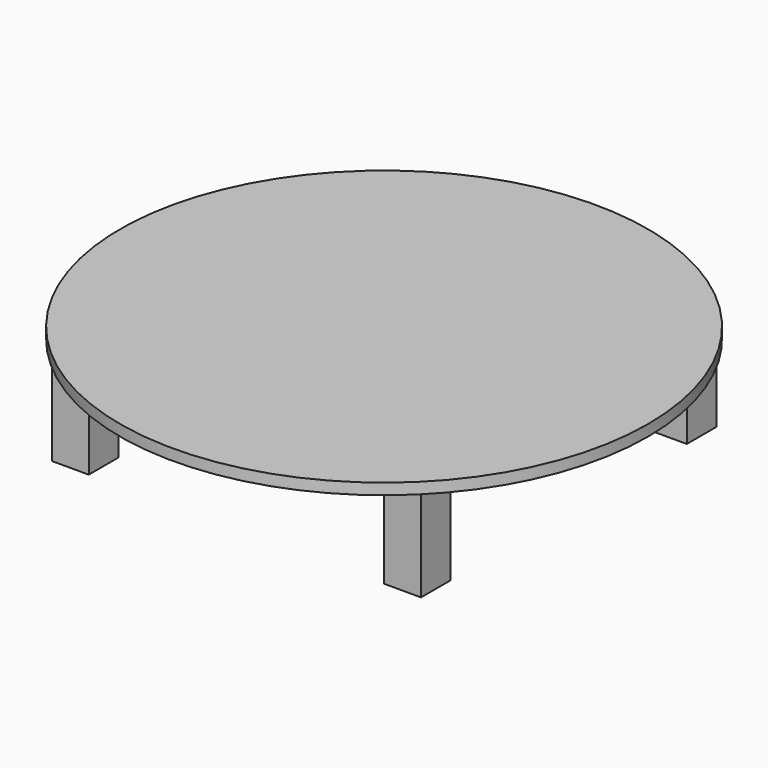
from build123d import *

# Parameters (mm, degrees)
F0_W     = 10
F0_H     = 10
F1_DEPTH = 25
F2_R     = 71.5
F3_DEPTH = 3
F6_R     = 70.6323523745
F7_DEPTH = 0.2


# Not quite as in the source:
# - the program builds the solid bodies; features that only make, move or delete a surface that nothing else refers to are left out


with BuildPart() as f1:
    # F0 (on Top) → F1 (new body)
    with BuildSketch(Plane.XY):
        with Locations((45, -45)):
            Rectangle(F0_W, F0_H)
    extrude(amount=F1_DEPTH)


with BuildPart() as f1b:
    # F0 (on Top) → F1, piece 2 (new body)
    with BuildSketch(Plane.XY):
        with Locations((45, 45)):
            Rectangle(F0_W, F0_H)
    extrude(amount=F1_DEPTH)


with BuildPart() as f1c:
    # F0 (on Top) → F1, piece 3 (new body)
    with BuildSketch(Plane.XY):
        with Locations((-45, -45)):
            Rectangle(F0_W, F0_H)
    extrude(amount=F1_DEPTH)


with BuildPart() as f1d:
    # F0 (on Top) → F1, piece 4 (new body)
    with BuildSketch(Plane.XY):
        with Locations((-45, 45)):
            Rectangle(F0_W, F0_H)
    extrude(amount=F1_DEPTH)


with BuildPart() as f3:
    # F2 (on face) → F3 (new body)
    with BuildSketch(Plane.XY.offset(25)):
        Circle(F2_R)
    extrude(amount=F3_DEPTH)


with BuildPart() as f7:
    # F6 (on face) → F7 (new body)
    with BuildSketch(Plane(origin=(0, 0, 25), x_dir=(1, 0, 0), z_dir=(0, 0, -1))):
        Circle(F6_R)
    extrude(amount=F7_DEPTH)


solid = Compound([f1.part, f1b.part, f1c.part, f1d.part, f3.part, f7.part])
